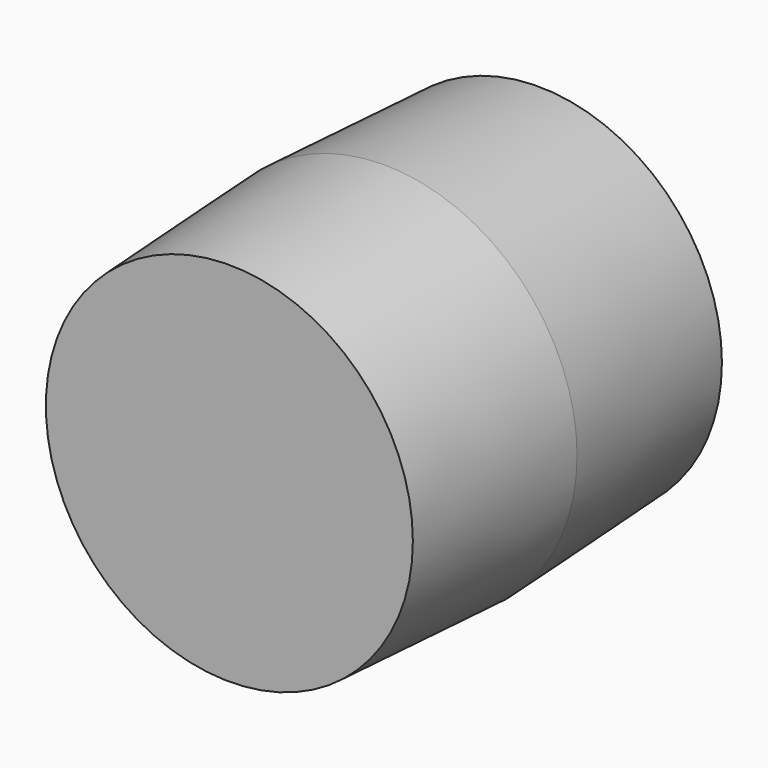
from build123d import *

# Parameters (mm, degrees)
F0_R     = 50.8
F1_DEPTH = 101.6
F2_SIZE2 = 2.53999
F2_SIZE  = 50.79999


# Not quite as in the source:
# - a fillet or chamfer is up to 0.001 mm smaller than in the source, because OpenCascade refuses the exact size


with BuildPart() as f1:
    # F0 (on Front) → F1 (new body)
    with BuildSketch(Plane.XZ):
        Circle(F0_R)
    extrude(amount=F1_DEPTH)

    # F2 (size 50.8 and 2.54 in the source; OpenCascade refuses exactly that, so slightly less here)
    f2_edges = [f1.edges().sort_by_distance(p)[0] for p in [
        (50.8, -50.8, 0),
        (-50.8, 0, 0),
        (-50.8, -101.6, 0),
    ]]
    chamfer(f2_edges, length=F2_SIZE, length2=F2_SIZE2)


solid = f1.part
